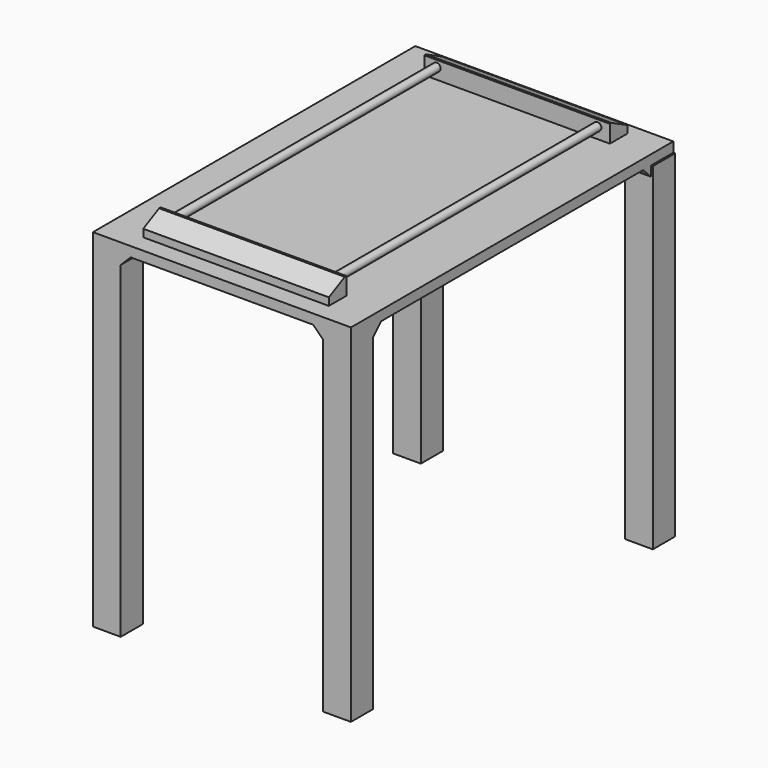
from build123d import *

# Parameters (mm, degrees)
F0_R      = 9.95
F7_DEPTH  = 55
F8_SIZE2  = 25
F8_SIZE   = 50
F10_W     = 650.0343084335
F10_H     = 1015.1521861553
F11_DEPTH = 25
F12_W     = 70
F12_H     = 70
F13_DEPTH = 850
F14_SIZE  = 25


with BuildPart() as f4:
    # F4: sweep along a path in F3
    with BuildLine(Plane.YZ.offset(-202.5484293699)) as f4_path:
        Line((-657.3717359189, -35.4168222417), (0, -35.4168222417))
        Line((0, -35.4168222417), (172.6282640811, -35.4168222417))
    # F0 (on Front) → F4 (sweep)
    with BuildSketch(Plane.XZ):
        with Locations((-202.5484293699, -35.1164080203)):
            Circle(F0_R)
    sweep(path=f4_path.line)


with BuildPart() as f5_1:
    # F5: instance of F4
    add(f4.part.mirror(Plane.YZ))


with BuildPart() as f7:
    # F6 (on face) → F7 (new body)
    with BuildSketch(Plane(origin=(0, 172.6282640811, 0), x_dir=(-1, 0, 0), z_dir=(0, 1, 0))):
        Polygon((0, -19.0347600728), (-233.8182926178, -19.0347600728), (-233.8182926178, -63.1103813648), (0, -63.1103813648), (233.8182926178, -63.1103813648), (233.8182926178, -19.0347600728), align=None)
    extrude(amount=F7_DEPTH)

    # F8
    f8_edges = [f7.edges().sort_by_distance(p)[0] for p in [
        (0, 227.628264, -19.03476),
    ]]
    f8_side = f7.faces().sort_by_distance((0, 200.128264, -19.03476))[0]
    chamfer(f8_edges, length=F8_SIZE, length2=F8_SIZE2, reference=f8_side)


with BuildPart() as f9_1:
    # F9: instance of F7
    add(f7.part.mirror(Plane.XZ.offset(242.372)))


with BuildPart() as f11:
    # F10 (on face) → F11 (new body)
    with BuildSketch(Plane(origin=(0, 0, -63.1103813648), x_dir=(1, 0, 0), z_dir=(0, 0, -1))):
        with Locations((0, 249.3127137423)):
            Rectangle(F10_W, F10_H)
    extrude(amount=F11_DEPTH)

    # F12 (on face) → F13 (join)
    with BuildSketch(Plane(origin=(0, 0, -88.1103813648), x_dir=(1, 0, 0), z_dir=(0, 0, -1))):
        with Locations((290.0171542168, 721.8888068199)):
            Rectangle(F12_W, F12_H)
        with Locations((294.588688612, -223.2633793354)):
            Rectangle(F12_W, F12_H)
        with Locations((-290.0171542168, -223.2633793354)):
            Rectangle(F12_W, F12_H)
        with Locations((-290.0171542168, 721.8888068199)):
            Rectangle(F12_W, F12_H)
    extrude(amount=F13_DEPTH)

    # F14
    f14_edges = [f11.edges().sort_by_distance(p)[0] for p in [
        (-255.017154, 223.263379, -88.110381),
        (-290.017154, 188.263379, -88.110381),
        (-255.017154, -721.888807, -88.110381),
        (292.302921, 188.263379, -88.110381),
        (259.588689, 223.263379, -88.110381),
        (255.017154, -721.888807, -88.110381),
        (290.017154, -686.888807, -88.110381),
        (-290.017154, -686.888807, -88.110381),
    ]]
    chamfer(f14_edges, length=F14_SIZE)


solid = Compound([f4.part, f5_1.part, f7.part, f9_1.part, f11.part])
